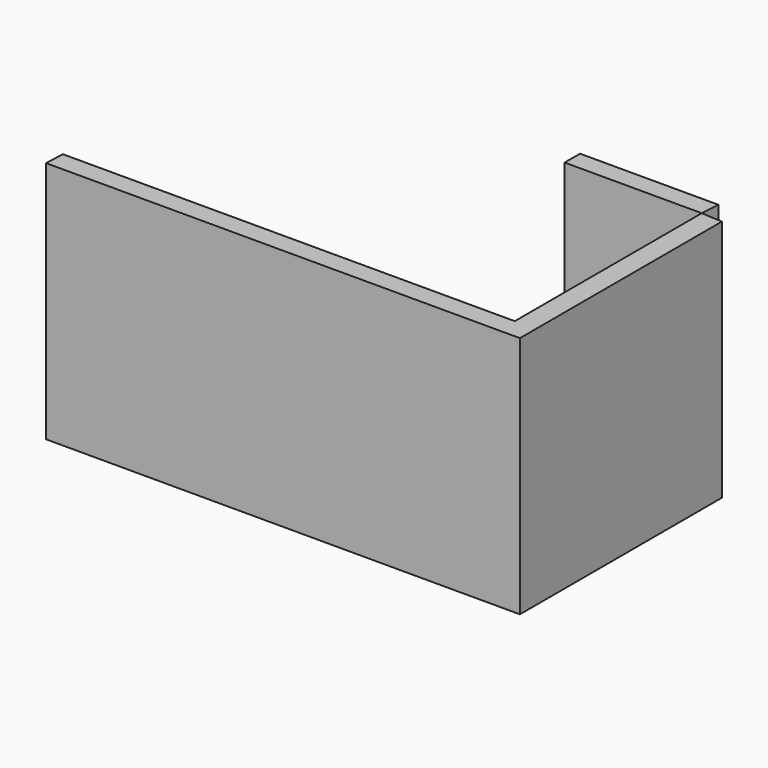
from build123d import *

# Parameters (mm, degrees)
F1_DEPTH = 44.45
F2_DEPTH = 43.688
F3_W     = 81.200633198
F3_H     = 3.012213856
F4_DEPTH = 11.938


# Not quite as in the source:
# - ends of sketch curves that miss each other by under 0.0002 mm in the source are joined


with BuildPart() as f1:
    # F0 (on Top) → F1 (new body)
    with BuildSketch(Plane.XY):
        Polygon((17.2227267176, 18.4892974794), (41.8306589127, 18.4892974794), (42.026810348, 21.9491124153), (17.1921476722, 21.9491124153), (17.1921476722, 18.4892974794), align=None)
    extrude(amount=-F1_DEPTH)


with BuildPart() as f2:
    # F0 (on Top) → F2 (new body)
    with BuildSketch(Plane.XY):
        Polygon((41.8306589127, -23.5073789954), (12.9724387079, -23.5073789954), (12.9724387079, -27.0969830453), (45.6240410119, -27.0969830453), (45.6240410119, 18.274234721), (41.8306589127, 18.4892974794), (41.8306589127, 10.6105906889), align=None)
        Polygon((-9.2982515926, -23.5073789954), (-39.3699742854, -23.5073789954), (-39.5123288035, -27.0969830453), (12.9724387079, -27.0969830453), (12.9724387079, -23.5073789954), align=None)
    extrude(amount=-F2_DEPTH)

    # F3 (on face) → F4 (join)
    with BuildSketch(Plane(origin=(0, -23.5073789954, 0), x_dir=(-1, 0, 0), z_dir=(0, 1, 0))):
        with Locations((-1.2303423136, -18.2796660811)):
            Rectangle(F3_W, F3_H)
    extrude(amount=F4_DEPTH)


solid = Compound([f1.part, f2.part])
